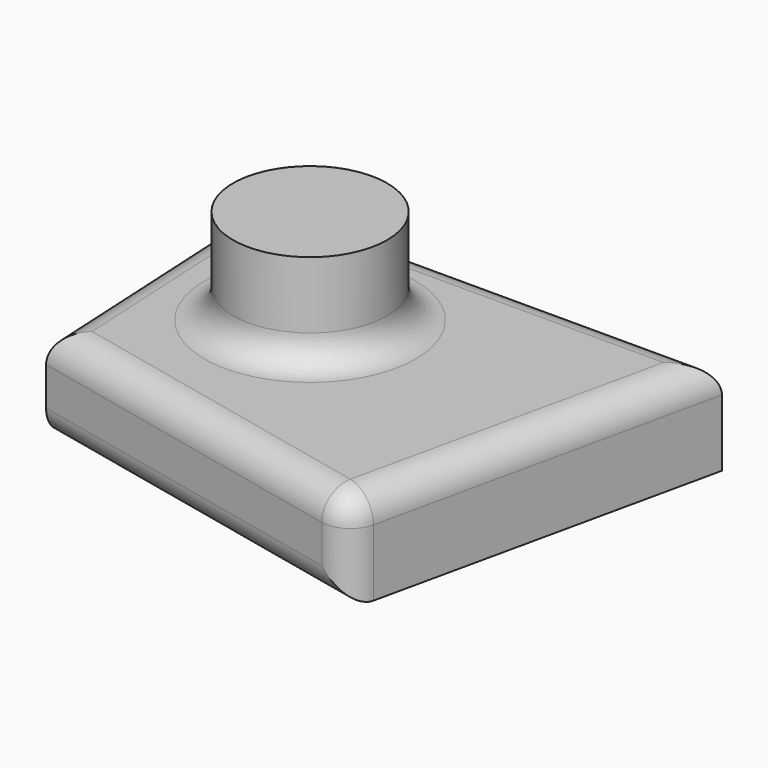
from build123d import *

# Parameters (mm, degrees)
F1_DEPTH = 25.4
F2_R     = 20.5214520654
F3_DEPTH = 25.4
F4_R     = 7.62


# Not quite as in the source:
# - the program builds the solid bodies; features that only make, move or delete a surface that nothing else refers to are left out


with BuildPart() as f1:
    # F0 (on Top) → F1 (new body)
    with BuildSketch(Plane.XY):
        Polygon((65.0288537145, 60.4610182345), (-57.2496131063, 60.4610182345), (-53.2582976497, -16.6874233163), (43.3438569307, -37.969596684), align=None)
    extrude(amount=F1_DEPTH)

    # F2 (on face) → F3 (join)
    with BuildSketch(Plane.XY.offset(25.4)):
        with Locations((-13.8034075499, 21.8867974591)):
            Circle(F2_R)
    extrude(amount=F3_DEPTH)

    # F4
    f4_edges = [f1.edges().sort_by_distance(p)[0] for p in [
        (54.186355, 11.245711, 25.4),
        (-4.95722, -27.32851, 25.4),
        (3.88962, 60.461018, 25.4),
        (-55.253955, 21.886797, 25.4),
        (-34.32486, 21.886797, 25.4),
        (43.343857, -37.969597, 12.7),
        (-4.95722, -27.32851, 0),
    ]]
    fillet(f4_edges, radius=F4_R)


solid = f1.part
